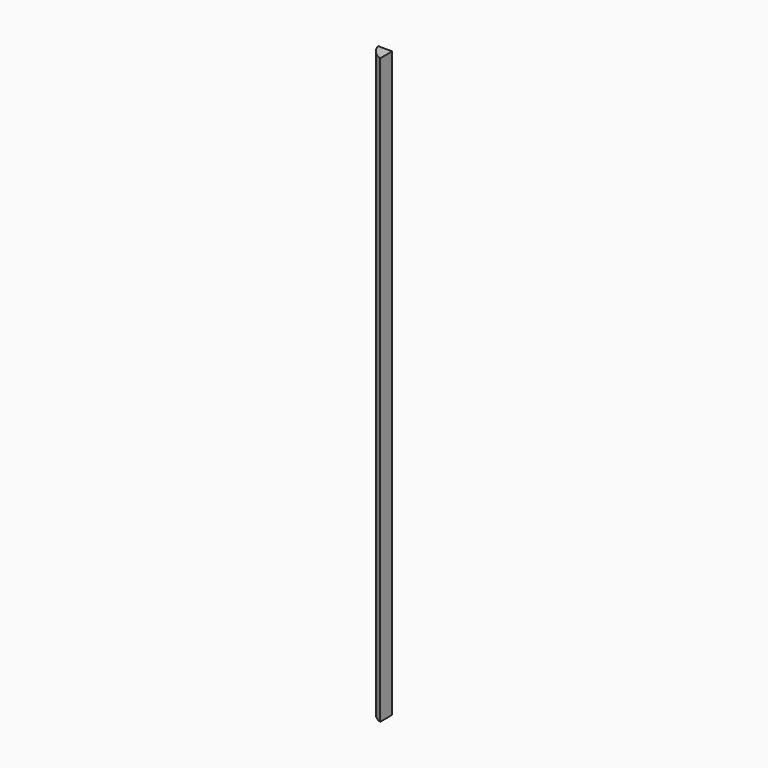
from build123d import *

# Parameters (mm, degrees)
F0_W        = 3.302
F0_H        = 3.302
F1_DEPTH    = 127
F2_T1_DEPTH = 150.7934423739


# Not quite as in the source:
# - a fillet or chamfer that OpenCascade refuses, or shapes differently, is made with other operations: its cross-section is extruded or revolved along the edge and cut away or added


with BuildPart() as f1:
    # F0 (on Top) → F1 (new body)
    with BuildSketch(Plane.XY):
        Rectangle(F0_W, F0_H)
    extrude(amount=F1_DEPTH)

    # F2: fillet of radius 5.08 on 1 edges, made by hand

    # F2_s2 → F2_t1 (cut)
    with BuildSketch(Plane.XY.offset(-11.8967211869)):
        with BuildLine():
            ThreePointArc((-1.651, 3.1076884748), (-0.7446458882, 0.211642895), (1.651, -1.651))
            Line((1.651, -1.651), (-1.651, -1.651))
            Line((-1.651, -1.651), (-1.651, 3.1076884748))
        make_face()
    extrude(amount=F2_T1_DEPTH, mode=Mode.SUBTRACT)


solid = f1.part
